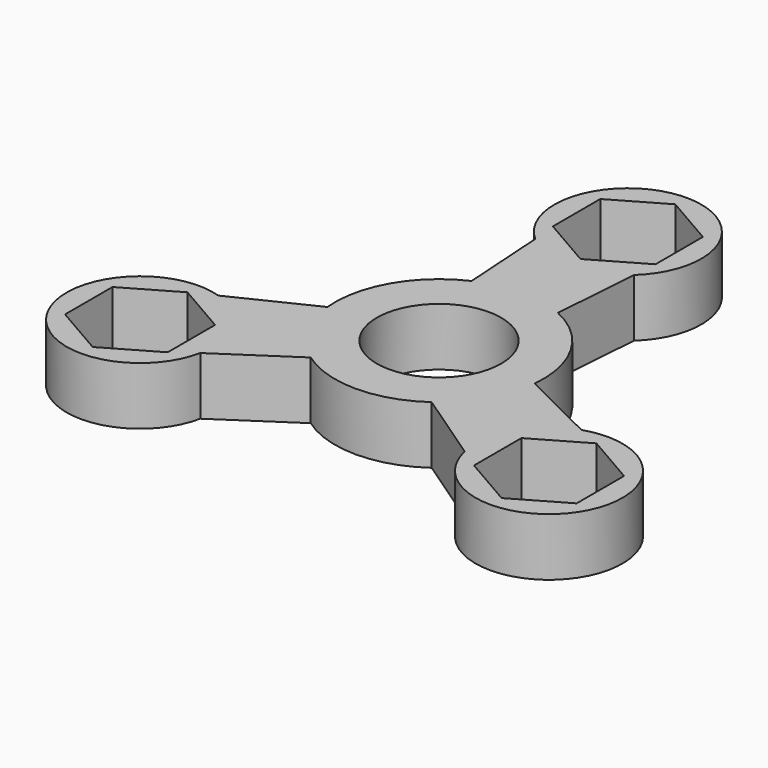
from build123d import *

# Parameters (mm, degrees)
F3_R     = 8.89
F1_R     = 12.6
F1_R_2   = 7.53
F5_DEPTH = 7
F6_DEPTH = 7
F0_R     = 7.53
F7_DEPTH = 7
F8_COUNT = 3


with BuildPart() as f5:
    # F3 (on Top) + F1 (on face) + F4 (on Top) → F5 (new body)
    with BuildSketch(Plane.XY):
        with Locations((0, 28.575)):
            Circle(F3_R)
    with BuildSketch(Plane.XY):
        Circle(F1_R)
        Circle(F1_R_2, mode=Mode.SUBTRACT)
    with BuildSketch(Plane.XY):
        Polygon((4.3963235803, 0), (6.1967625508, 24.9068178236), (-6.0855683336, 24.9068178236), (-4.4936764197, 0), align=None)
    extrude(amount=F5_DEPTH)

    # F2 (on Top) → F6 (cut)
    with BuildSketch(Plane.XY):
        Polygon((6.21, 24.9896548283), (6.21, 32.1603451717), (0, 35.7456903433), (-6.21, 32.1603451717), (-6.21, 24.9896548283), (0, 21.4043096567), align=None)
    extrude(amount=F6_DEPTH, mode=Mode.SUBTRACT)

    # F0 (on Top) → F7 (cut)
    with BuildSketch(Plane.XY):
        Circle(F0_R)
    extrude(amount=F7_DEPTH, mode=Mode.SUBTRACT)

    # F8: F5 ×3 about axis
    f8_axis = Axis((0, 0, 7), (0, 0, -1))


with BuildPart() as f5_1:
    add(f5.part)
    for i in range(1, F8_COUNT):
        add(f5.part.rotate(f8_axis, i * 360 / F8_COUNT))


solid = f5_1.part
